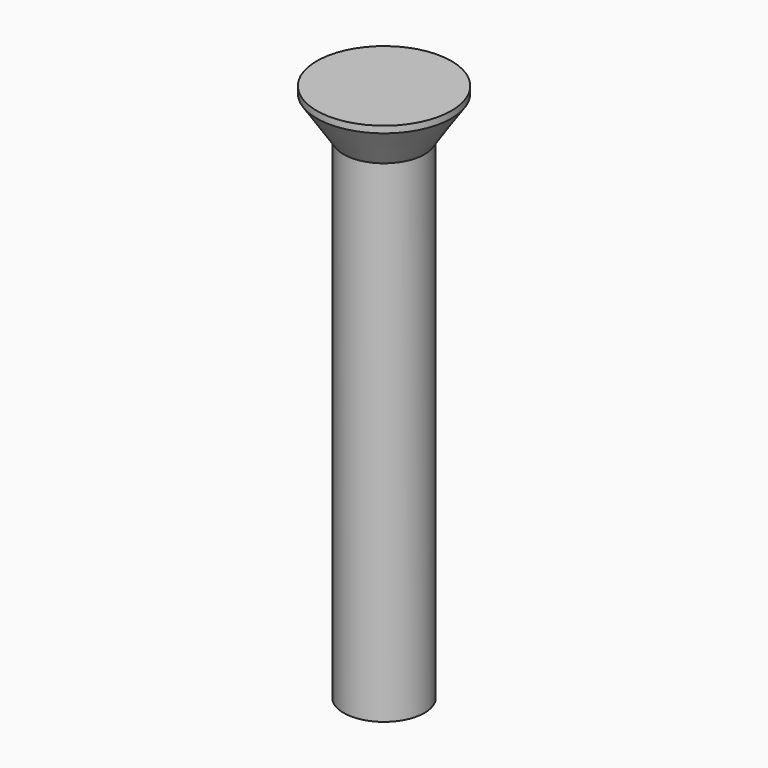
from build123d import *

# Parameters (mm, degrees)
F0_R     = 5
F1_DEPTH = 3.5
F2_R     = 3
F3_DEPTH = 36.5
F4_SIZE2 = 1.99999
F4_SIZE  = 2.99999


# Not quite as in the source:
# - a fillet or chamfer is up to 0.001 mm smaller than in the source, because OpenCascade refuses the exact size


with BuildPart() as f1:
    # F0 (on Top) → F1 (new body)
    with BuildSketch(Plane.XY):
        Circle(F0_R)
    extrude(amount=F1_DEPTH)

    # F2 (on face) → F3 (join)
    with BuildSketch(Plane(origin=(0, 0, 0), x_dir=(1, 0, 0), z_dir=(0, 0, -1))):
        Circle(F2_R)
    extrude(amount=F3_DEPTH)

    # F4 (size 3 and 2 in the source; OpenCascade refuses exactly that, so slightly less here)
    f4_edges = [f1.edges().sort_by_distance(p)[0] for p in [
        (-5, 0, 0),
    ]]
    f4_side = f1.faces().sort_by_distance((-5, 0, 1.75))[0]
    chamfer(f4_edges, length=F4_SIZE, length2=F4_SIZE2, reference=f4_side)


solid = f1.part
